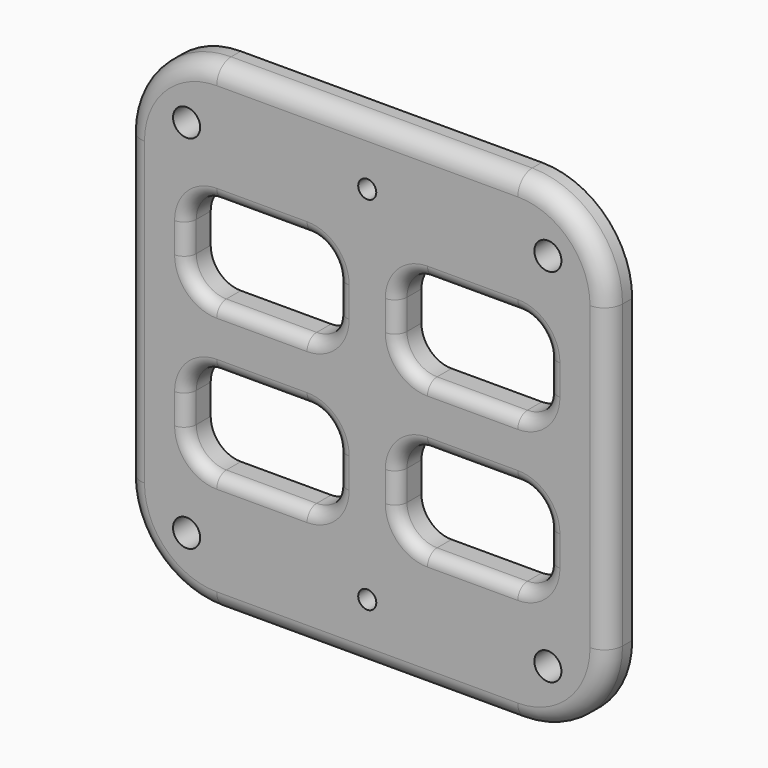
from build123d import *

# Parameters (mm, degrees)
F0_W     = 80
F0_H     = 80
F0_R     = 2.25
F0_W_2   = 25
F0_H_2   = 15
F0_R_2   = 1.5
F1_DEPTH = 5
F2_R     = 5
F3_R     = 5
F4_R     = 5
F5_R     = 15
F6_R     = 3
F7_R     = 2
F8_R     = 3.5
F9_DEPTH = 2


with BuildPart() as f1:
    # F0 (on Front) → F1 (new body)
    with BuildSketch(Plane.XZ):
        Rectangle(F0_W, F0_H)
        with Locations((-30, -30)):
            Circle(F0_R, mode=Mode.SUBTRACT)
        with Locations((-17.5, -12.5)):
            Rectangle(F0_W_2, F0_H_2, mode=Mode.SUBTRACT)
        with Locations((0, -30)):
            Circle(F0_R_2, mode=Mode.SUBTRACT)
        with Locations((30, -30)):
            Circle(F0_R, mode=Mode.SUBTRACT)
        with Locations((17.5, -12.5)):
            Rectangle(F0_W_2, F0_H_2, mode=Mode.SUBTRACT)
        with Locations((-17.5, 12.5)):
            Rectangle(F0_W_2, F0_H_2, mode=Mode.SUBTRACT)
        with Locations((-30, 30)):
            Circle(F0_R, mode=Mode.SUBTRACT)
        with Locations((17.5, 12.5)):
            Rectangle(F0_W_2, F0_H_2, mode=Mode.SUBTRACT)
        with Locations((0, 30)):
            Circle(F0_R_2, mode=Mode.SUBTRACT)
        with Locations((30, 30)):
            Circle(F0_R, mode=Mode.SUBTRACT)
    extrude(amount=F1_DEPTH)

    # F2
    f2_edges = [f1.edges().sort_by_distance(p)[0] for p in [
        (30, -2.5, 5),
        (30, -2.5, 20),
        (5, -2.5, 20),
        (5, -2.5, 5),
    ]]
    fillet(f2_edges, radius=F2_R)

    # F3
    f3_edges = [f1.edges().sort_by_distance(p)[0] for p in [
        (-30, -2.5, 20),
        (-30, -2.5, 5),
        (-5, -2.5, 5),
        (-5, -2.5, 20),
    ]]
    fillet(f3_edges, radius=F3_R)

    # F4
    f4_edges = [f1.edges().sort_by_distance(p)[0] for p in [
        (-5, -2.5, -5),
        (30, -2.5, -5),
        (5, -2.5, -5),
        (-30, -2.5, -5),
        (30, -2.5, -20),
        (-5, -2.5, -20),
        (5, -2.5, -20),
        (-30, -2.5, -20),
    ]]
    fillet(f4_edges, radius=F4_R)

    # F5
    f5_edges = [f1.edges().sort_by_distance(p)[0] for p in [
        (40, -2.5, -40),
        (40, -2.5, 40),
        (-40, -2.5, 40),
        (-40, -2.5, -40),
    ]]
    fillet(f5_edges, radius=F5_R)

    # F6
    f6_edges = [f1.edges().sort_by_distance(p)[0] for p in [
        (35.606602, -5, 35.606602),
    ]]
    fillet(f6_edges, radius=F6_R)

    # F7
    f7_edges = [f1.edges().sort_by_distance(p)[0] for p in [
        (6.464466, -5, 18.535534),
        (6.464466, -5, -6.464466),
        (-28.535534, -5, 18.535534),
        (-28.535534, -5, -6.464466),
    ]]
    fillet(f7_edges, radius=F7_R)

    # F8 (on face) → F9 (cut)
    with BuildSketch(Plane(origin=(0, 0, 0), x_dir=(-1, 0, 0), z_dir=(0, 1, 0))):
        with Locations((0, 30)):
            Circle(F8_R)
        with Locations((0, -30)):
            Circle(F8_R)
    extrude(amount=-F9_DEPTH, mode=Mode.SUBTRACT)


solid = f1.part
